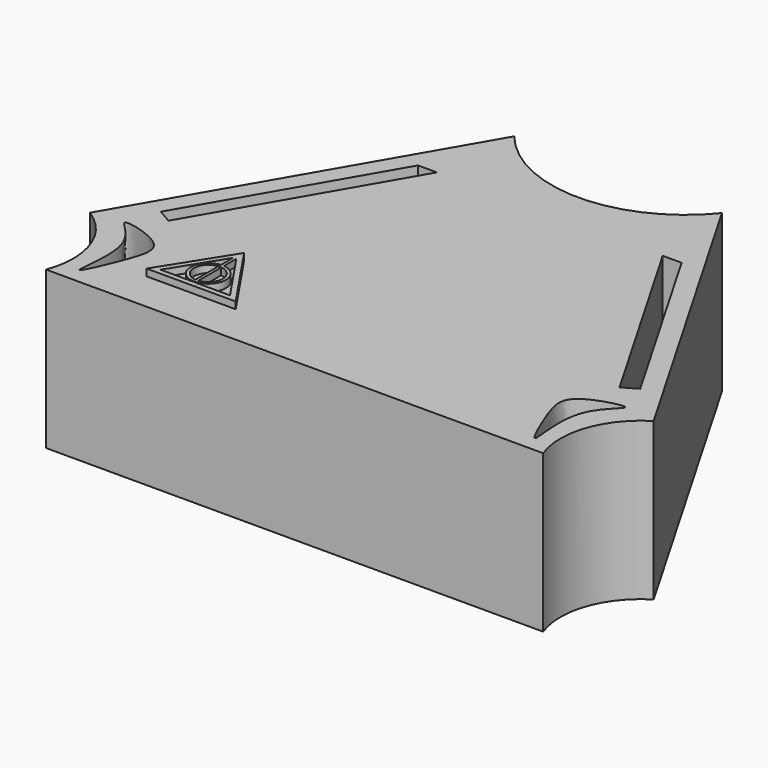
from build123d import *

# Parameters (mm, degrees)
F1_DEPTH    = 12.192
F2_T        = 2.54
F2_T3_DEPTH = 17.272
F3_R        = 8.6389696703
F3_R_2      = 7.1951480733
F4_DEPTH    = 7.62
F6_DEPTH    = 0.5334
F8_DEPTH    = 0.5334
F9_R        = 1.3596518107
F9_R_2      = 1.1254343815
F10_DEPTH   = 0.5588


# Not quite as in the source:
# - a shell that OpenCascade refuses in one call is made with other operations: the cavity is built on its own and cut out


with BuildPart() as f1:
    # F0 (on Top) → F1 (new body)
    with BuildSketch(Plane.XY):
        with BuildLine():
            Line((-19.2829854786, -24.7512944043), (0, -24.7512944043))
            Line((0, -24.7512944043), (19.2829854786, -24.7512944043))
            ThreePointArc((19.2829854786, -24.7512944043), (19.2425419625, -20.5475069912), (21.8732375652, -17.2683447599))
            Line((21.8732375652, -17.2683447599), (8.0585619435, 6.6195321269))
            ThreePointArc((8.0585619435, 6.6195321269), (0, 2.7777536427), (-8.0585619435, 6.6195321269))
            Line((-8.0585619435, 6.6195321269), (-21.8732375652, -17.2683447599))
            ThreePointArc((-21.8732375652, -17.2683447599), (-19.2425419625, -20.5475069912), (-19.2829854786, -24.7512944043))
        make_face()
        with BuildLine():
            add(Edge.make_bspline(
                [(-19.3815156817, -16.9240329415), (-19.5938714539, -17.0906957951), (-16.7265937937, -18.7842348459), (-18.3822608443, -25.6109655406), (-16.1081655346, -20.3388174448), (-15.4053597577, -17.6966909211), (-19.151813561, -16.7437561798), (-19.3815156817, -16.9240329415)],
                knots=[0, 0, 0, 0, 0.184075193, 0.4179305813, 0.6185874945, 0.8008885665, 1, 1, 1, 1], degree=3))
        make_face(mode=Mode.SUBTRACT)
        with BuildLine():
            add(Edge.make_bspline(
                [(19.3815156817, -16.9240329415), (19.5938714539, -17.0906957951), (16.7265937937, -18.7842348459), (18.3822608443, -25.6109655406), (16.1081655346, -20.3388174448), (15.4053597577, -17.6966909211), (19.151813561, -16.7437561798), (19.3815156817, -16.9240329415)],
                knots=[0, 0, 0, 0, 0.184075193, 0.4179305813, 0.6185874945, 0.8008885665, 1, 1, 1, 1], degree=3))
        make_face(mode=Mode.SUBTRACT)
        Polygon((-18.5983052961, -14.4770355546), (-10.2260438725, 0), (-8.7601219289, 0), (-17.4997807305, -15.1123268619), align=None, mode=Mode.SUBTRACT)
        Polygon((18.5983052961, -14.4770355546), (17.4997807305, -15.1123268619), (8.7601219289, 0), (10.2260438725, 0), align=None, mode=Mode.SUBTRACT)
    extrude(amount=F1_DEPTH)

    # F2: shell of thickness 2.54, made by hand


with BuildPart() as f2_core1:
    # F2_t2: copy of F1
    add(f1.part)

    # the walls: a layer under each face that stays
    f2_faces = [f2_core1.faces().sort_by_distance(p)[0] for p in [
        (-19.2425419625, -20.5475069912, 6.096),
        (0, -9.4957167068, 12.192),
        (9.4930829007, 0, 6.096),
        (13.1299513297, -7.5561634309, 6.096),
        (18.0490430133, -14.7946812082, 6.096),
        (14.4121745843, -7.2385177773, 6.096),
        (-13.1299513297, -7.5561634309, 6.096),
        (-9.4930829007, 0, 6.096),
        (-14.4121745843, -7.2385177773, 6.096),
        (-18.0490430133, -14.7946812082, 6.096),
        (17.2482511109, -22.877015161, 6.096),
        (-17.2482511109, -22.877015161, 6.096),
        (0, 2.7777536427, 6.096),
        (14.9658997543, -5.3244063165, 6.096),
        (19.2425419625, -20.5475069912, 6.096),
        (0, -24.7512944043, 6.096),
        (-14.9658997543, -5.3244063165, 6.096),
    ]]
    thicken(f2_faces, amount=-F2_T, mode=Mode.SUBTRACT)

    # F2_s4 → F2_t3 (cut)
    with BuildSketch(Plane.XY.offset(-2.54)):
        Polygon((8.7821097999, -0.012684123), (8.7601219289, 2.54), (4.3570431715, 2.54), (6.5613348293, -1.2715877047), align=None)
        Polygon((10.2040560015, -0.038115877), (10.2260438725, 2.54), (11.6912913404, 2.54), (12.4248309721, 1.2715877047), align=None)
        Polygon((17.5090527244, -15.0776231138), (15.3009936309, -16.3839145666), (16.5725813357, -18.5827016661), (18.7713684352, -17.3111139614), align=None)
        Polygon((18.563601548, -14.4677635606), (19.8698930008, -16.6758226541), (22.0686801004, -15.4042349494), (20.7970923956, -13.2054478498), align=None)
        Polygon((-8.7821097999, -0.012684123), (-6.5613348293, -1.2715877047), (-4.3570431715, 2.54), (-8.7601219289, 2.54), align=None)
        Polygon((-17.5090527244, -15.0776231138), (-15.3009936309, -16.3839145666), (-16.5725813357, -18.5827016661), (-18.7713684352, -17.3111139614), align=None)
        Polygon((-10.2040560015, -0.038115877), (-10.2260438725, 2.54), (-11.6912913404, 2.54), (-12.4248309721, 1.2715877047), align=None)
        Polygon((-18.563601548, -14.4677635606), (-20.7970923956, -13.2054478498), (-22.0686801004, -15.4042349494), (-19.8698930008, -16.6758226541), align=None)
    extrude(amount=F2_T3_DEPTH, mode=Mode.SUBTRACT)


with BuildPart() as f1_1:
    add(f1.part)

    # what is left inside the walls is the cavity
    f2_cavity = [f2_core1.part.solids().sort_by_distance(p)[0] for p in [
        (0, -14.380477, 9.6266),
        (-7.421374, 2.5654, 6.434667),
        (7.421374, 2.5654, 6.434667),
    ]]
    add(f2_cavity, mode=Mode.SUBTRACT)

    # F3 (on face) → F4 (join)
    with BuildSketch(Plane(origin=(0, 0, 9.652), x_dir=(1, 0, 0), z_dir=(0, 0, -1))):
        with Locations((0, 10.6488130987)):
            Circle(F3_R)
        with Locations((-2.6933e-06, 10.6488130987)):
            Circle(F3_R_2, mode=Mode.SUBTRACT)
    extrude(amount=F4_DEPTH)

    # F5 (on face) → F6 (join)
    with BuildSketch(Plane.XY.offset(12.192)):
        Polygon((-7.0586228797, -21.6420597119), (-10.6374602765, -16.3539252019), (-13.9745017514, -21.6420597119), align=None)
        Polygon((-13.2216994964, -21.2318077683), (-10.6374602765, -17.0818977058), (-7.8289361557, -21.2318077683), align=None, mode=Mode.SUBTRACT)
    extrude(amount=F6_DEPTH)

    # F7 (on face) → F8 (join)
    with BuildSketch(Plane.XY.offset(12.192)):
        Polygon((-10.5269337073, -17.0413207984), (-10.753906332, -17.0413207984), (-10.753906332, -21.2964676321), (-10.5269337073, -21.4800376163), align=None)
    extrude(amount=F8_DEPTH)

    # F9 (on face) → F10 (join)
    with BuildSketch(Plane.XY.offset(12.192)):
        with Locations((-10.6177497655, -19.846925512)):
            Circle(F9_R)
        with Locations((-10.6177497655, -19.846925512)):
            Circle(F9_R_2, mode=Mode.SUBTRACT)
    extrude(amount=F10_DEPTH)


solid = f1_1.part
